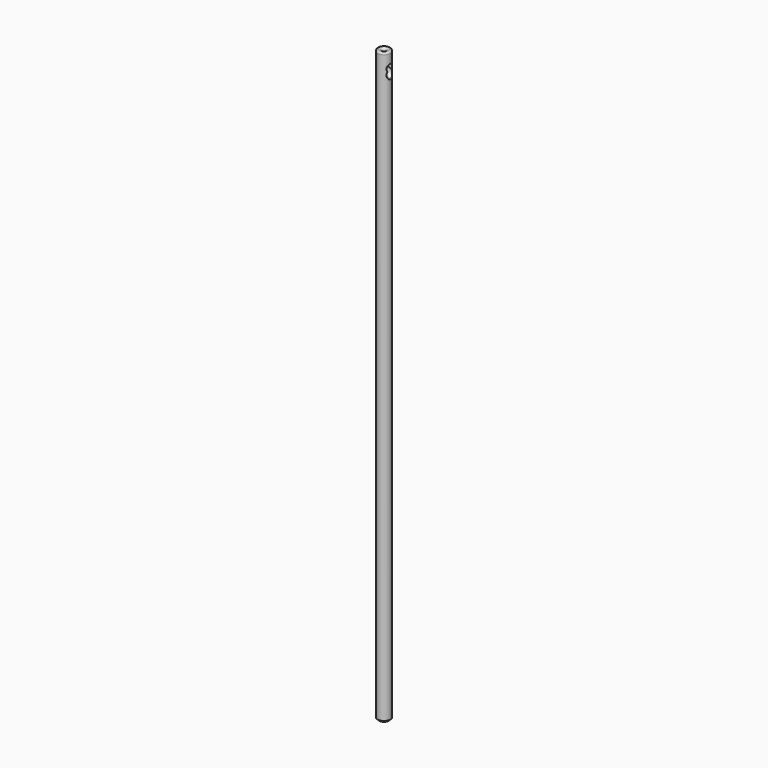
from build123d import *
from build123d import SkipClean  # not in build123d's __all__


with BuildPart() as f1:
    # F0 (on Front) → F1 (revolve)
    with BuildSketch(Plane.XZ):
        with BuildLine():
            Line((-3.5, 324), (-3.5, 1))
            Line((-3.5, 1), (-2.5, 0))
            Line((-2.5, 0), (0, 0))
            Line((0, 0), (0, 317.4226497308))
            Line((0, 317.4226497308), (-1, 318))
            Line((-1, 318), (-1, 323.5))
            ThreePointArc((-1, 323.5), (-1.4393398282, 324.5606601718), (-2.5, 325))
            ThreePointArc((-2.5, 325), (-3.2071067812, 324.7071067812), (-3.5, 324))
        make_face()
    revolve(axis=Axis((0, 0, 158.7113248654), (0, 0, -1)))

    # F2 (on Front) → F3 (revolve, cut)
    with BuildSketch(Plane.XZ):
        Polygon((-1, 319), (-2.1547005384, 317), (10.5847728806, 317), (10.5847728806, 319), align=None)
    revolve(axis=Axis((7.4317818913, 0, 317), (1, 0, 0)), mode=Mode.SUBTRACT)

    # F4 (on Front) → F5 (revolve, cut)
    with BuildSketch(Plane.XZ):
        Polygon((7.5055534995, 311.4226497308), (1.3094010768, 315), (-1, 315), (-1, 316.3333333333), (-2.1547005384, 317), (-2.1547005384, 314.6905989232), (6.5055534995, 309.6905989232), align=None)
        Polygon((-1, 315), (1.3094010768, 315), (-1, 316.3333333333), align=None)
    with SkipClean():  # cleaning this boolean's faces spoils the solid; the shape is the same uncleaned
        revolve(axis=Axis((2.6754264805, 0, 314.2113248654), (0.8660254038, 0, -0.5)), mode=Mode.SUBTRACT)


solid = f1.part
